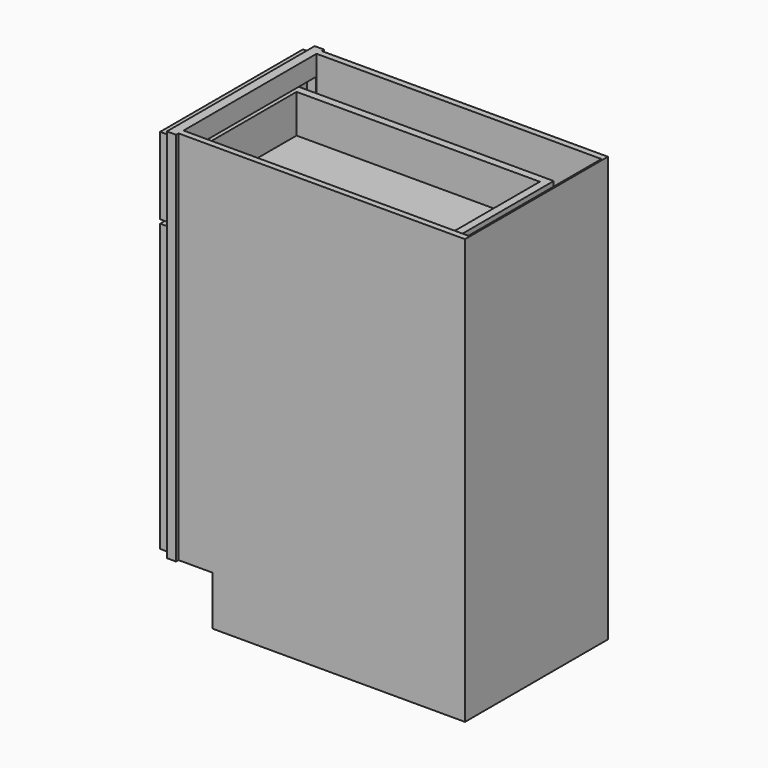
from build123d import *

# Parameters (mm, degrees)
F0_W          = 609.6
F0_H          = 876.3
F1_DEPTH      = 381
F2_W          = 88.9
F2_H          = 101.6
F3_DEPTH      = 381.001
F4_W          = 340.4016393443
F4_H          = 692.15
F5_DEPTH      = 19.05
F6_W          = 590.55
F6_H          = 6.35
F7_DEPTH      = 876.301
F8_W          = 587.375
F8_H          = 342.9
F9_DEPTH      = 733.425
F10_W         = 340.4016393443
F10_H         = 41.275
F11_DEPTH     = 19.05
F12_W         = 368.3
F12_H         = 590.5627
F12_W_2       = 254
F12_H_2       = 476.2627
F13_DEPTH     = 19.05
F14_W         = 6.35
F14_H         = 254
F15_DEPTH     = 476.2627
F16_SIZE      = 3.175
F17_W         = 368.3
F17_H         = 158.75
F17_W_2       = 254
F17_H_2       = 82.55
F18_DEPTH     = 19.05
F19_W         = 6.35
F19_H         = 254
F20_DEPTH     = 82.55
F21_SIZE      = 3.175
F22_W         = 504.825
F22_H         = 342.9
F23_DEPTH     = 101.6
F24_W         = 279.4
F24_H         = 95.25
F25_DEPTH     = 533.4
F26_T         = 15.875
F26_T3_DEPTH  = 37.249261314
F26_T5_DEPTH  = 37.249261314
F26_T7_DEPTH  = 37.249261314
F26_T9_DEPTH  = 37.249261314
F26_T11_DEPTH = 36.5125
F26_T13_DEPTH = 285.75
F26_T15_DEPTH = 114.3
F26_T17_DEPTH = 127
F26_T19_DEPTH = 311.15
F26_T21_DEPTH = 111.125
F26_T23_DEPTH = 36.5125


# Not quite as in the source:
# - a shell that OpenCascade refuses in one call is made with other operations: the cavity is built on its own and cut out


with BuildPart() as f1:
    # F0 (on Front) → F1 (new body)
    with BuildSketch(Plane.XZ):
        Rectangle(F0_W, F0_H)
    extrude(amount=-F1_DEPTH)

    # F2 (on face) → F3 (cut, through all)
    with BuildSketch(Plane.XZ):
        with Locations((-260.35, -387.35)):
            Rectangle(F2_W, F2_H)
    extrude(amount=-F3_DEPTH, mode=Mode.SUBTRACT)

    # F4 (on face) → F5 (cut)
    with BuildSketch(Plane(origin=(-304.8, 0, 0), x_dir=(0, -1, 0), z_dir=(-1, 0, 0))):
        with Locations((-190.5, 50.8)):
            Rectangle(F4_W, F4_H)
    extrude(amount=-F5_DEPTH, mode=Mode.SUBTRACT)

    # F6 (on face) → F7 (cut, through all)
    with BuildSketch(Plane.XY.offset(438.15)):
        with Locations((9.525, 377.825)):
            Rectangle(F6_W, F6_H)
        with Locations((9.525, 3.175)):
            Rectangle(F6_W, F6_H)
    extrude(amount=-F7_DEPTH, mode=Mode.SUBTRACT)

    # F8 (on face) → F9 (cut, through all)
    with BuildSketch(Plane.XY.offset(438.15)):
        with Locations((7.9375, 190.5)):
            Rectangle(F8_W, F8_H)
    extrude(amount=-F9_DEPTH, mode=Mode.SUBTRACT)

    # F10 (on face) → F11 (join, through all)
    with BuildSketch(Plane(origin=(-304.8, 0, 0), x_dir=(0, -1, 0), z_dir=(-1, 0, 0))):
        with Locations((-190.5, 265.1125)):
            Rectangle(F10_W, F10_H)
    extrude(amount=-F11_DEPTH)

    # F22 (on face) → F23 (cut)
    with BuildSketch(Plane(origin=(0, 0, -438.15), x_dir=(1, 0, 0), z_dir=(0, 0, -1))):
        with Locations((49.2125, -190.5)):
            Rectangle(F22_W, F22_H)
    extrude(amount=-F23_DEPTH, mode=Mode.SUBTRACT)


with BuildPart() as f13:
    # F12 (on face) → F13 (new body)
    with BuildSketch(Plane(origin=(-304.8, 0, 0), x_dir=(0, -1, 0), z_dir=(-1, 0, 0))):
        with Locations((-190.5, -33.33115)):
            Rectangle(F12_W, F12_H)
        with Locations((-190.5, -33.33115)):
            Rectangle(F12_W_2, F12_H_2, mode=Mode.SUBTRACT)
    extrude(amount=F13_DEPTH)

    # F14 (on face) → F15 (join, through all)
    with BuildSketch(Plane.XY.offset(-271.4625)):
        with Locations((-312.7375, 190.5)):
            Rectangle(F14_W, F14_H)
    extrude(amount=F15_DEPTH)

    # F16
    f16_edges = [f13.edges().sort_by_distance(p)[0] for p in [
        (-323.85, 317.5, -33.33115),
        (-323.85, 190.5, -271.4625),
        (-323.85, 63.5, -33.33115),
        (-323.85, 190.5, 204.8002),
    ]]
    chamfer(f16_edges, length=F16_SIZE)


with BuildPart() as f18:
    # F17 (on face) → F18 (new body)
    with BuildSketch(Plane(origin=(-304.8, 0, 0), x_dir=(0, -1, 0), z_dir=(-1, 0, 0))):
        with Locations((-190.5, 349.25)):
            Rectangle(F17_W, F17_H)
        with Locations((-190.5, 349.25)):
            Rectangle(F17_W_2, F17_H_2, mode=Mode.SUBTRACT)
    extrude(amount=F18_DEPTH)

    # F19 (on face) → F20 (join, through all)
    with BuildSketch(Plane.XY.offset(307.975)):
        with Locations((-312.7375, 190.5)):
            Rectangle(F19_W, F19_H)
    extrude(amount=F20_DEPTH)

    # F21
    f21_edges = [f18.edges().sort_by_distance(p)[0] for p in [
        (-323.85, 190.5, 307.975),
        (-323.85, 317.5, 349.25),
        (-323.85, 190.5, 390.525),
        (-323.85, 63.5, 349.25),
    ]]
    chamfer(f21_edges, length=F21_SIZE)

    # F24 (on face) → F25 (join)
    with BuildSketch(Plane.YZ.offset(-304.8)):
        with Locations((190.5, 339.725)):
            Rectangle(F24_W, F24_H)
    extrude(amount=F25_DEPTH)

    # F26: shell of thickness 15.875, made by hand


with BuildPart() as f26_core1:
    # F26_t2: copy of F18
    add(f18.part)

    # the walls: a layer under each face that stays
    f26_faces = [f26_core1.faces().sort_by_distance(p)[0] for p in [
        (-323.85, 313.2666666667, 296.3333333333),
        (-322.2625, 190.5, 306.3875),
        (-322.2625, 61.9125, 349.25),
        (-322.2625, 319.0875, 349.25),
        (-322.2625, 190.5, 392.1125),
        (-314.325, 190.5, 428.625),
        (-314.325, 374.65, 349.25),
        (-314.325, 190.5, 269.875),
        (-314.325, 6.35, 349.25),
        (-318.29375, 190.5, 307.975),
        (-318.29375, 63.5, 349.25),
        (-318.29375, 317.5, 349.25),
        (-318.29375, 190.5, 390.525),
        (-304.8, 313.2666666667, 402.1666666667),
        (-315.9125, 190.5, 349.25),
        (-38.1, 330.2, 339.725),
        (-38.1, 190.5, 292.1),
        (-38.1, 50.8, 339.725),
        (-307.18125, 63.5, 349.25),
        (-307.18125, 190.5, 390.525),
        (-307.18125, 317.5, 349.25),
        (-304.8, 190.5, 347.6625),
        (228.6, 190.5, 339.725),
        (-307.18125, 190.5, 307.975),
        (-309.5625, 190.5, 349.25),
    ]]
    thicken(f26_faces, amount=-F26_T, mode=Mode.SUBTRACT)

    # F26_s4 → F26_t3 (cut)
    with BuildSketch(Plane(origin=(4.5928978099, 4.5928978099, 4.5928978099), x_dir=(-0.7071067812, 0.7071067812, 0), z_dir=(0.5773502692, 0.5773502692, 0.5773502692))):
        Polygon((271.8908726623, 356.5892701441), (263.7152476623, 342.7036353262), (255.7777476623, 347.2863530879), (255.7777476623, 356.4517886113), align=None)
    extrude(amount=F26_T3_DEPTH, mode=Mode.SUBTRACT)

    # F26_s6 → F26_t5 (cut)
    with BuildSketch(Plane(origin=(-122.4071021901, 122.4071021901, -122.4071021901), x_dir=(0.7071067812, 0.7071067812, 0), z_dir=(0.5773502692, -0.5773502692, 0.5773502692))):
        Polygon((-2.4831890303, 512.1318688108), (5.6924359697, 498.2462339929), (13.6299359697, 502.8289517546), (13.6299359697, 511.994387278), align=None)
    extrude(amount=F26_T5_DEPTH, mode=Mode.SUBTRACT)

    # F26_s8 → F26_t7 (cut)
    with BuildSketch(Plane(origin=(-228.2404355234, -228.2404355234, 228.2404355234), x_dir=(-0.7071067812, 0.7071067812, 0), z_dir=(0.5773502692, 0.5773502692, -0.5773502692))):
        Polygon((271.8908726623, 213.7335916339), (255.7777476623, 213.8710731668), (255.7777476623, 223.0365086901), (263.7152476623, 227.6192264518), align=None)
    extrude(amount=F26_T7_DEPTH, mode=Mode.SUBTRACT)

    # F26_s10 → F26_t9 (cut)
    with BuildSketch(Plane(origin=(-355.2404355234, 355.2404355234, 355.2404355234), x_dir=(0.7071067812, 0.7071067812, 0), z_dir=(0.5773502692, -0.5773502692, -0.5773502692))):
        Polygon((-2.4831890303, 58.1909929672), (13.6299359697, 58.3284745), (13.6299359697, 67.4939100234), (5.6924359697, 72.0766277851), align=None)
    extrude(amount=F26_T9_DEPTH, mode=Mode.SUBTRACT)

    # F26_s12 → F26_t11 (cut)
    with BuildSketch(Plane.YZ.offset(-336.55)):
        Polygon((317.34125, 308.13375), (317.5, 292.1), (333.375, 292.1), (333.375, 307.975), align=None)
        Polygon((63.65875, 308.13375), (63.5, 292.1), (47.625, 292.1), (47.625, 307.975), align=None)
        Polygon((63.65875, 390.36625), (47.625, 390.525), (47.625, 406.4), (63.5, 406.4), align=None)
        Polygon((317.34125, 390.36625), (333.375, 390.525), (333.375, 406.4), (317.5, 406.4), align=None)
    extrude(amount=F26_T11_DEPTH, mode=Mode.SUBTRACT)

    # F26_s14 → F26_t13 (cut)
    with BuildSketch(Plane.XZ.offset(-333.375)):
        Polygon((-316.07125, 308.13375), (-315.9125, 292.1), (-300.0375, 292.1), (-300.0375, 307.975), align=None)
        Polygon((-316.07125, 390.36625), (-315.9125, 406.4), (-300.0375, 406.4), (-300.0375, 390.525), align=None)
        Polygon((-309.40375, 390.36625), (-309.5625, 406.4), (-325.4375, 406.4), (-325.4375, 390.525), align=None)
        Polygon((-304.95875, 308.13375), (-288.925, 307.975), (-288.925, 292.1), (-304.8, 292.1), align=None)
        Polygon((-309.40375, 308.13375), (-309.5625, 292.1), (-325.4375, 292.1), (-325.4375, 307.975), align=None)
    extrude(amount=F26_T13_DEPTH, mode=Mode.SUBTRACT)

    # F26_s16 → F26_t15 (cut)
    with BuildSketch(Plane.XY.offset(292.1)):
        Polygon((-316.07125, 63.65875), (-315.9125, 47.625), (-300.0375, 47.625), (-300.0375, 63.5), align=None)
        Polygon((-316.07125, 317.34125), (-315.9125, 333.375), (-300.0375, 333.375), (-300.0375, 317.5), align=None)
        Polygon((-309.40375, 63.65875), (-309.5625, 47.625), (-325.4375, 47.625), (-325.4375, 63.5), align=None)
        Polygon((-309.40375, 317.34125), (-309.5625, 333.375), (-325.4375, 333.375), (-325.4375, 317.5), align=None)
    extrude(amount=F26_T15_DEPTH, mode=Mode.SUBTRACT)

    # F26_s18 → F26_t17 (cut)
    with BuildSketch(Plane.XY.offset(276.225)):
        Polygon((-304.64125, 330.35875), (-320.675, 330.2), (-320.675, 314.325), (-304.8, 314.325), align=None)
        Polygon((-304.64125, 50.64125), (-320.675, 50.8), (-320.675, 66.675), (-304.8, 66.675), align=None)
    extrude(amount=F26_T17_DEPTH, mode=Mode.SUBTRACT)

    # F26_s20 → F26_t19 (cut)
    with BuildSketch(Plane.XZ.offset(-346.075)):
        Polygon((-304.64125, 291.94125), (-320.675, 292.1), (-320.675, 307.975), (-304.8, 307.975), align=None)
    extrude(amount=F26_T19_DEPTH, mode=Mode.SUBTRACT)

    # F26_s22 → F26_t21 (cut)
    with BuildSketch(Plane.XY.offset(292.1)):
        Polygon((-304.95875, 63.65875), (-304.8, 47.625), (-288.925, 47.625), (-288.925, 63.5), align=None)
        Polygon((-304.95875, 317.34125), (-304.8, 333.375), (-288.925, 333.375), (-288.925, 317.5), align=None)
    extrude(amount=F26_T21_DEPTH, mode=Mode.SUBTRACT)

    # F26_s24 → F26_t23 (cut)
    with BuildSketch(Plane.YZ.offset(-325.4375)):
        Polygon((63.65875, 308.13375), (47.625, 307.975), (47.625, 292.1), (63.5, 292.1), align=None)
        Polygon((63.65875, 390.36625), (47.625, 390.525), (47.625, 406.4), (63.5, 406.4), align=None)
        Polygon((317.34125, 390.36625), (317.5, 406.4), (333.375, 406.4), (333.375, 390.525), align=None)
        Polygon((317.34125, 308.13375), (333.375, 307.975), (333.375, 292.1), (317.5, 292.1), align=None)
    extrude(amount=F26_T23_DEPTH, mode=Mode.SUBTRACT)


with BuildPart() as f18_1:
    add(f18.part)

    # what is left inside the walls is the cavity
    f26_cavity = [f26_core1.part.solids().sort_by_distance(p)[0] for p in [
        (45.508333, 190.5, 308.13375),
    ]]
    add(f26_cavity, mode=Mode.SUBTRACT)


solid = Compound([f1.part, f13.part, f18_1.part])
